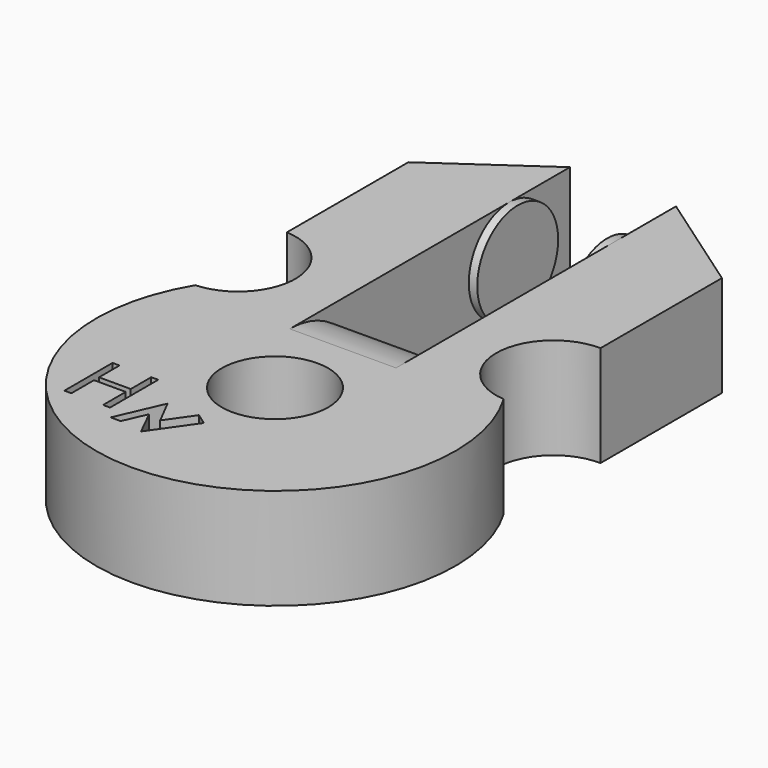
from build123d import *

# Parameters (mm, degrees)
F0_R         = 3.15
F1_DEPTH     = 6
F2_T4_DEPTH  = 33.7860809536
F2_T10_DEPTH = 33.7860809536
F3_R         = 3
F4_DEPTH     = 7
F5_TEXT_SIZE = 4.9978908565
F6_DEPTH     = 25
F8_W         = 7.3854723014
F8_H         = 8.5189908277
F9_DEPTH     = 5.3


# Not quite as in the source:
# - a fillet or chamfer that OpenCascade refuses, or shapes differently, is made with other operations: its cross-section is extruded or revolved along the edge and cut away or added
# - Text() gives the source's letters only with a copy of the font that has no kerning and outlines rounded to 1/6400 em; it was checked with that copy


with BuildPart() as f1:
    # F0 (on Top) → F1 (new body)
    with BuildSketch(Plane.XY):
        with BuildLine():
            Line((3.1341714785, -13.3385833821), (3.1341714785, -20.9635833821))
            Line((3.1341714785, -20.9635833821), (-3.1518919859, -20.9784116596))
            Line((-3.1518919859, -20.9784116596), (-3.1518919859, -13.2135833821))
            Line((-3.1518919859, -13.2135833821), (-3.1518919859, -7.2135833821))
            Line((-3.1518919859, -7.2135833821), (-3.1518919859, -5.7135833821))
            Line((-3.1518919859, -5.7135833821), (-9.3052557186, -10.0014866894))
            Line((-9.3052557186, -10.0014866894), (-9.3052557186, -19.0014866894))
            ThreePointArc((-9.3052557186, -19.0014866894), (-6.0826153167, -22.396857593), (-9.3052557186, -25.7922284966))
            ThreePointArc((-9.3052557186, -25.7922284966), (-0.161923888, -41.9031792413), (8.9814079425, -25.7922284966))
            ThreePointArc((8.9814079425, -25.7922284966), (5.8274290148, -22.2477758085), (9.2875352111, -19.0014866894))
            Line((9.2875352111, -19.0014866894), (9.2875352111, -10.0014866894))
            Line((9.2875352111, -10.0014866894), (3.1341714785, -5.7135833821))
            Line((3.1341714785, -5.7135833821), (3.1341714785, -7.2135833821))
            Line((3.1341714785, -7.2135833821), (3.1341714785, -13.3385833821))
        make_face()
        with Locations((0, -31.515585149)):
            Circle(F0_R, mode=Mode.SUBTRACT)
    extrude(amount=F1_DEPTH)

    # F2: fillet of radius 5.5 on 2 edges, made by hand


with BuildPart() as f2_tool2:
    # F2_s3 → F2_t4 (new body)
    with BuildSketch(Plane(origin=(16.8346647865, 0.0397115114, 0), x_dir=(0, 0, 1), z_dir=(-0.9999972178, -0.0023589065, 0))):
        with BuildLine():
            ThreePointArc((0.5, -20.9709182743), (4.3890872965, -22.5818309778), (6, -26.4709182743))
            Line((6, -26.4709182743), (6.11, -26.4709182743))
            Line((6.11, -26.4709182743), (6.11, -20.8609182743))
            Line((6.11, -20.8609182743), (0.5, -20.8609182743))
            Line((0.5, -20.8609182743), (0.5, -20.9709182743))
        make_face()
    extrude(amount=F2_T4_DEPTH)

    split(bisect_by=Plane.YZ.offset(3.1341714785), keep=Keep.BOTTOM)

    split(bisect_by=Plane.YZ.offset(-3.1518919859), keep=Keep.TOP)


with BuildPart() as f1_1:
    add(f1.part)

    # F2_t1: cut F2_tool2
    add(f2_tool2.part, mode=Mode.SUBTRACT)


with BuildPart() as f2_tool8:
    # F2_s9 → F2_t10 (new body)
    with BuildSketch(Plane(origin=(16.8346647865, 0.0397115114, 0), x_dir=(0, 0, 1), z_dir=(-0.9999972178, -0.0023589065, 0))):
        with BuildLine():
            ThreePointArc((5.5, -20.9709182743), (1.6109127035, -22.5818309778), (0, -26.4709182743))
            Line((0, -26.4709182743), (-0.11, -26.4709182743))
            Line((-0.11, -26.4709182743), (-0.11, -20.8609182743))
            Line((-0.11, -20.8609182743), (5.5, -20.8609182743))
            Line((5.5, -20.8609182743), (5.5, -20.9709182743))
        make_face()
    extrude(amount=F2_T10_DEPTH)

    split(bisect_by=Plane.YZ.offset(3.1341714785), keep=Keep.BOTTOM)

    split(bisect_by=Plane.YZ.offset(-3.1518919859), keep=Keep.TOP)


with BuildPart() as f1_2:
    add(f1_1.part)

    # F2_t7: cut F2_tool8
    add(f2_tool8.part, mode=Mode.SUBTRACT)

    # F3 (on face) → F4 (join)
    with BuildSketch(Plane.YZ.offset(-3.1518919859)):
        with Locations((-10.2135833821, 3)):
            Circle(F3_R)
    extrude(amount=F4_DEPTH)

    # F5 (on face) → F6 (cut)
    with BuildSketch(Plane.XY.offset(6)):
        Polygon((-2.8923563659, -35.8603447676), (-4.0845102631, -38.5889559984), (-3.4884333145, -38.5889559984), (-2.8923563659, -37.224650383), (-2.1062763408, -38.8148711008), (-0.364724441, -36.3293362251), (-1.034066896, -35.8603447676), (-2.1062763408, -37.3905971646), align=None)
        with Locations((-7.9209171236, -37.8358736634)):
            Text('H', F5_TEXT_SIZE, font='Open Sans', text_align=(TextAlign.LEFT, TextAlign.BOTTOM))
    extrude(amount=-F6_DEPTH, mode=Mode.SUBTRACT)

    # F8 (on offset) → F9 (cut)
    with BuildSketch(Plane.YZ.offset(-2.6518919859)):
        with Locations((-10.2746502962, 2.4762806715)):
            Rectangle(F8_W, F8_H)
    extrude(amount=F9_DEPTH, mode=Mode.SUBTRACT)


solid = f1_2.part
